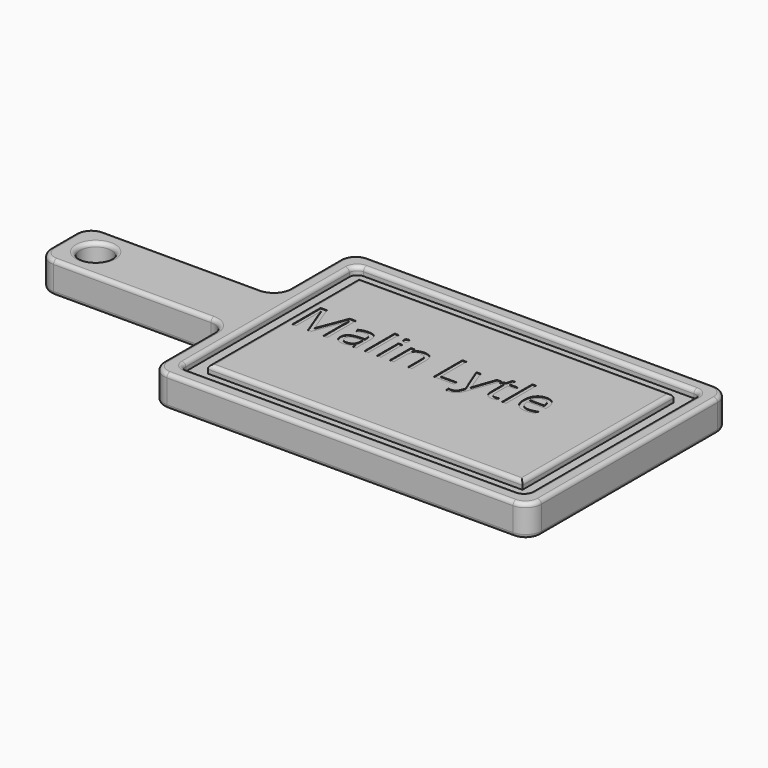
from build123d import *

# Parameters (mm, degrees)
F0_W         = 152.4
F0_H         = 50.8
F1_DEPTH     = 25.4
F2_R         = 12.7
F3_DEPTH     = 25.4
F5_DEPTH     = 6.35
F6_R         = 6.35
F7_R         = 12.7
F8_R         = 3.175
F9_TEXT_SIZE = 40.3099621846
F10_DEPTH    = 0.508


# Not quite as in the source:
# - Text() gives the source's letters only with a copy of the font that has no kerning and outlines rounded to 1/6400 em; it was checked with that copy


with BuildPart() as f1:
    # F0 (on Top) → F1 (new body)
    with BuildSketch(Plane.XY):
        Polygon((0, 76.2), (0, 0), (304.8, 0), (304.8, 203.2), (0, 203.2), (0, 127), align=None)
        with Locations((-76.2, 101.6)):
            Rectangle(F0_W, F0_H)
    extrude(amount=F1_DEPTH)

    # F2 (on face) → F3 (cut)
    with BuildSketch(Plane.XY.offset(25.4)):
        with Locations((-126.0605752468, 101.6)):
            Circle(F2_R)
    extrude(amount=-F3_DEPTH, mode=Mode.SUBTRACT)

    # F4 (on face) → F5 (cut)
    with BuildSketch(Plane.XY.offset(25.4)):
        Polygon((12.6999939203, 76.2), (12.6999939203, 12.6999939203), (292.1000060797, 12.6999939203), (292.1000060797, 190.5000060797), (12.6999939203, 190.5000060797), (12.6999939203, 127), align=None)
        Polygon((25.4000002861, 76.2), (25.4000002861, 127), (25.4000002861, 177.7999997139), (279.3999997139, 177.7999997139), (279.3999997139, 25.4000002861), (25.4000002861, 25.4000002861), align=None, mode=Mode.SUBTRACT)
    extrude(amount=-F5_DEPTH, mode=Mode.SUBTRACT)

    # F6
    f6_edges = [f1.edges().sort_by_distance(p)[0] for p in [
        (12.699994, 190.500006, 22.225),
        (292.100006, 190.500006, 22.225),
        (12.699994, 12.699994, 22.225),
        (292.100006, 12.699994, 22.225),
    ]]
    fillet(f6_edges, radius=F6_R)

    # F7
    f7_edges = [f1.edges().sort_by_distance(p)[0] for p in [
        (-152.4, 76.2, 12.7),
        (-152.4, 127, 12.7),
        (0, 76.2, 12.7),
        (0, 0, 12.7),
        (304.8, 0, 12.7),
        (0, 203.2, 12.7),
        (304.8, 203.2, 12.7),
        (0, 127, 12.7),
    ]]
    fillet(f7_edges, radius=F7_R)

    # F8
    f8_edges = [f1.edges().sort_by_distance(p)[0] for p in [
        (152.4, 177.8, 25.4),
        (279.4, 101.6, 25.4),
        (152.4, 25.4, 25.4),
        (25.4, 101.6, 25.4),
        (0, 38.1, 25.4),
        (-3.719744, 72.480256, 25.4),
        (3.719744, 3.719744, 25.4),
        (-76.2, 76.2, 25.4),
        (152.4, 0, 25.4),
        (-148.680256, 79.919744, 25.4),
        (301.080256, 3.719744, 25.4),
        (-152.4, 101.6, 25.4),
        (304.8, 101.6, 25.4),
        (-148.680256, 123.280256, 25.4),
        (301.080256, 199.480256, 25.4),
        (-76.2, 127, 25.4),
        (152.4, 203.2, 25.4),
        (-3.719744, 130.719744, 25.4),
        (3.719744, 199.480256, 25.4),
        (0, 165.1, 25.4),
        (152.4, 12.699994, 25.4),
        (14.559866, 14.559866, 25.4),
        (290.240134, 14.559866, 25.4),
        (12.699994, 101.6, 25.4),
        (292.100006, 101.6, 25.4),
        (14.559866, 188.640134, 25.4),
        (290.240134, 188.640134, 25.4),
        (152.4, 190.500006, 25.4),
        (-138.760575, 101.6, 25.4),
        (0, 38.1, 0),
        (-3.719744, 72.480256, 0),
        (3.719744, 3.719744, 0),
        (-76.2, 76.2, 0),
        (152.4, 0, 0),
        (-148.680256, 79.919744, 0),
        (301.080256, 3.719744, 0),
        (-152.4, 101.6, 0),
        (304.8, 101.6, 0),
        (-148.680256, 123.280256, 0),
        (301.080256, 199.480256, 0),
        (-76.2, 127, 0),
        (152.4, 203.2, 0),
        (-3.719744, 130.719744, 0),
        (3.719744, 199.480256, 0),
        (0, 165.1, 0),
        (-138.760575, 101.6, 0),
    ]]
    fillet(f8_edges, radius=F8_R)

    # F9 (on face) → F10 (cut)
    with BuildSketch(Plane.XY.offset(25.4)):
        with Locations((28.5750002861, 101.6)):
            Text('Malin Lytle', F9_TEXT_SIZE, font='Open Sans', text_align=(TextAlign.LEFT, TextAlign.BOTTOM))
    extrude(amount=-F10_DEPTH, mode=Mode.SUBTRACT)


solid = f1.part
